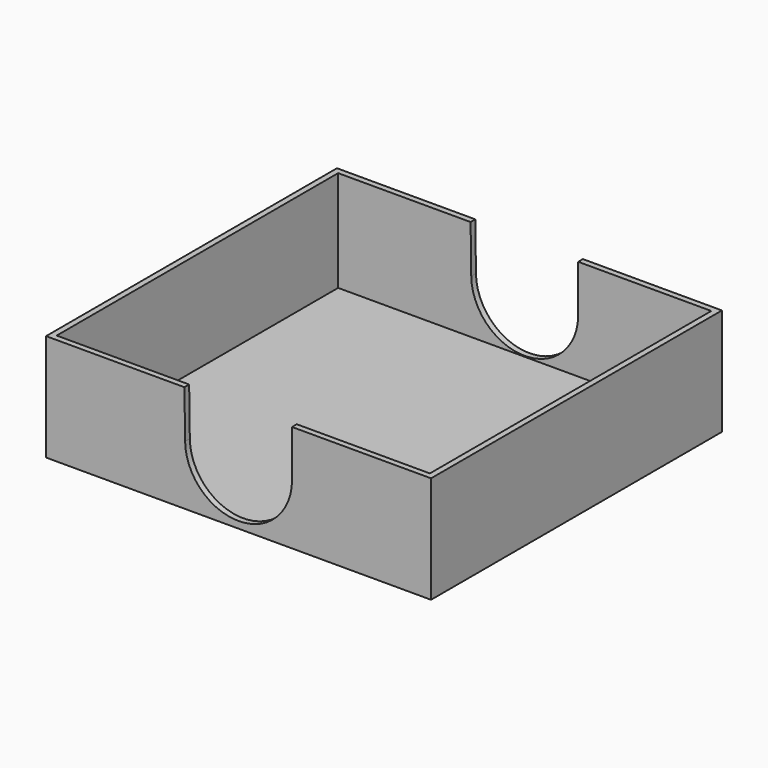
from build123d import *

# Parameters (mm, degrees)
F0_W     = 114.3
F0_H     = 107.95
F1_DEPTH = 31.75
F3_T     = -1.75
F4_DEPTH = 1.75


# Not quite as in the source:
# - a pattern or mirror of a feature is missing from the dataset's text; its kind, count and spacing are read off the source's solid


with BuildPart() as f1:
    # F0 (on Top) → F1 (new body)
    with BuildSketch(Plane.XY):
        Rectangle(F0_W, F0_H)
    extrude(amount=F1_DEPTH)

    # F3
    f3_openings = [f1.faces().sort_by_distance(p)[0] for p in [
        (0, 0, 31.75),
    ]]
    offset(amount=F3_T, openings=f3_openings)

    # F2 (on face) → F4 (cut)
    with BuildSketch(Plane.XZ.offset(53.975)):
        with BuildLine():
            ThreePointArc((-7.7136243103, 31.75), (-13.7391570489, 25.8280615857), (-15.873456613, 17.6536402154))
            ThreePointArc((-15.873456613, 17.6536402154), (0, 2), (15.873456613, 17.6536402154))
            Line((15.873456613, 17.6536402154), (15.873456613, 18.0963597846))
            ThreePointArc((15.873456613, 18.0963597846), (13.6269244294, 26.0188661333), (7.7136243103, 31.75))
            Line((7.7136243103, 31.75), (-7.7136243103, 31.75))
        make_face()
        with BuildLine():
            Line((-16.0700342862, 31.75), (-15.873456613, 17.6536402154))
            ThreePointArc((-15.873456613, 17.6536402154), (-13.7391570489, 25.8280615857), (-7.7136243103, 31.75))
            Line((-7.7136243103, 31.75), (-16.0700342862, 31.75))
        make_face()
        with BuildLine():
            Line((15.873456613, 18.0963597846), (15.873456613, 17.6536402154))
            ThreePointArc((15.873456613, 17.6536402154), (15.8746141486, 17.7643174175), (15.875, 17.875))
            ThreePointArc((15.875, 17.875), (15.8746141486, 17.9856825825), (15.873456613, 18.0963597846))
        make_face()
        with BuildLine():
            ThreePointArc((7.7136243103, 31.75), (0, 33.75), (-7.7136243103, 31.75))
            Line((-7.7136243103, 31.75), (7.7136243103, 31.75))
        make_face()
        with BuildLine():
            ThreePointArc((7.7136243103, 31.75), (13.6269244294, 26.0188661333), (15.873456613, 18.0963597846))
            Line((15.873456613, 18.0963597846), (15.873456613, 31.75))
            Line((15.873456613, 31.75), (7.7136243103, 31.75))
        make_face()
    f4 = extrude(amount=-F4_DEPTH, mode=Mode.SUBTRACT)

    # F4_copies: F4 across plane
    add(f4.mirror(Plane.ZX), mode=Mode.SUBTRACT)


solid = f1.part
